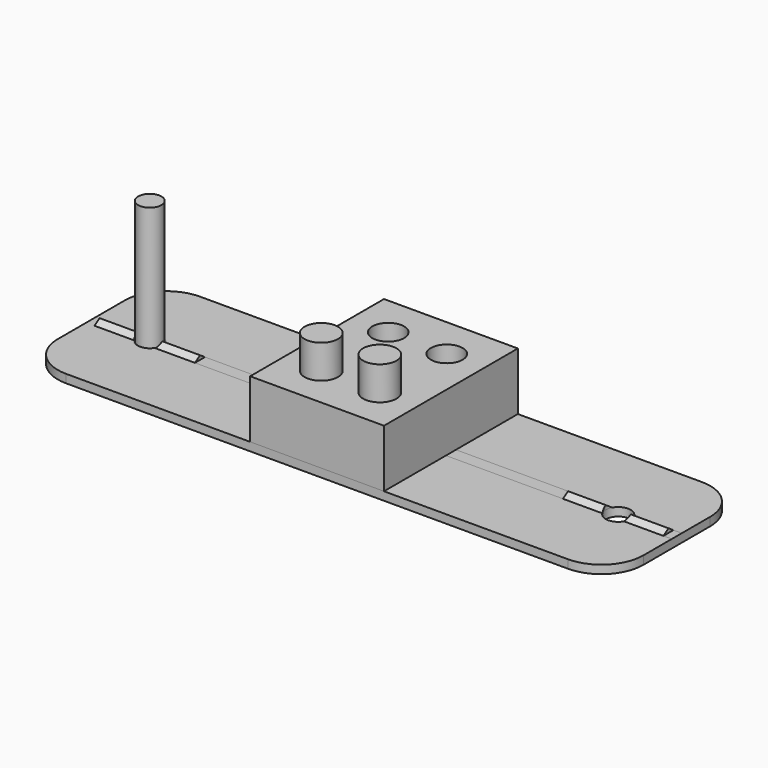
from build123d import *
from build123d import SkipClean  # not in build123d's __all__

# Parameters (mm, degrees)
F0_W      = 70
F0_H      = 20
F1_DEPTH  = 1
F3_D      = 3
F4_R      = 5
F7_DEPTH  = 0.5
F9_DEPTH  = 69.001
F10_W     = 16
F10_H     = 9.25
F10_H_2   = 1.5
F11_DEPTH = 6.9
F12_R     = 1.9
F13_DEPTH = 4.5
F14_R     = 2
F15_DEPTH = 4
F16_R     = 1.5
F17_DEPTH = 1
F18_R     = 1.4
F19_DEPTH = 14.8


with BuildPart() as f1:
    # F0 (on Top) → F1 (new body)
    with BuildSketch(Plane.XY):
        Rectangle(F0_W, F0_H)
    extrude(amount=F1_DEPTH)

    # F3 (through all)
    with Locations(Plane.XY.offset(1)):
        with Locations((-28, 0), (28, 0)):
            Hole(F3_D / 2)

    # F4
    f4_edges = [f1.edges().sort_by_distance(p)[0] for p in [
        (-35, 10, 0.5),
        (-35, -10, 0.5),
        (35, 10, 0.5),
        (35, -10, 0.5),
    ]]
    fillet(f4_edges, radius=F4_R)

    # F5 (on face) + F6 (on face) → F7 (join)
    with BuildSketch(Plane.XY.offset(1)):
        with BuildLine():
            Line((-29.2990381057, 0.75), (-34, 0.75))
            Line((-34, 0.75), (-34, -0.75))
            Line((-34, -0.75), (-29.2990381057, -0.75))
            ThreePointArc((-29.2990381057, -0.75), (-29.5, 0), (-29.2990381057, 0.75))
        make_face()
        with BuildLine():
            Line((-22, 0.75), (-26.7009618943, 0.75))
            ThreePointArc((-26.7009618943, 0.75), (-26.5511112606, 0.3882285677), (-26.5, 0))
            ThreePointArc((-26.5, 0), (-26.5511112606, -0.3882285677), (-26.7009618943, -0.75))
            Line((-26.7009618943, -0.75), (-22, -0.75))
            Line((-22, -0.75), (-22, 0.75))
        make_face()
    with BuildSketch(Plane.XY.offset(1)):
        with BuildLine():
            Line((26.7009618943, 0.75), (22, 0.75))
            Line((22, 0.75), (22, -0.75))
            Line((22, -0.75), (26.7009618943, -0.75))
            ThreePointArc((26.7009618943, -0.75), (26.5, 0), (26.7009618943, 0.75))
        make_face()
        with BuildLine():
            Line((34, 0.75), (29.2990381057, 0.75))
            ThreePointArc((29.2990381057, 0.75), (29.4488887394, 0.3882285677), (29.5, 0))
            ThreePointArc((29.5, 0), (29.4488887394, -0.3882285677), (29.2990381057, -0.75))
            Line((29.2990381057, -0.75), (34, -0.75))
            Line((34, -0.75), (34, 0.75))
        make_face()
    with SkipClean():  # cleaning this boolean's faces spoils the solid; the shape is the same uncleaned
        extrude(amount=F7_DEPTH)

    # F8 (on face) → F9 (cut, through all)
    with BuildSketch(Plane(origin=(-34, 0, 0), x_dir=(0, -1, 0), z_dir=(-1, 0, 0))):
        Polygon((-0.75, 1.5), (-0.75, 1), (0, 1.5), align=None)
        Polygon((0.75, 1.5), (0, 1.5), (0.75, 1), align=None)
    with SkipClean():  # cleaning this boolean's faces spoils the solid; the shape is the same uncleaned
        extrude(amount=-F9_DEPTH, mode=Mode.SUBTRACT)

    # F10 (on face) → F11 (join)
    with BuildSketch(Plane.XY.offset(1)):
        with Locations((0, -5.375)):
            Rectangle(F10_W, F10_H)
        Rectangle(F10_W, F10_H_2)
        with Locations((0, 5.375)):
            Rectangle(F10_W, F10_H)
    with SkipClean():  # cleaning this boolean's faces spoils the solid; the shape is the same uncleaned
        extrude(amount=F11_DEPTH)

    # F12 (on face) → F13 (cut)
    with BuildSketch(Plane.XY.offset(7.9)):
        with Locations((-3.5, 5)):
            Circle(F12_R)
        with Locations((3.5, 5)):
            Circle(F12_R)
    with SkipClean():  # cleaning this boolean's faces spoils the solid; the shape is the same uncleaned
        extrude(amount=-F13_DEPTH, mode=Mode.SUBTRACT)

    # F14 (on face) → F15 (join)
    with BuildSketch(Plane.XY.offset(7.9)):
        with Locations((-3.5, -5)):
            Circle(F14_R)
        with Locations((3.5, -5)):
            Circle(F14_R)
    with SkipClean():  # cleaning this boolean's faces spoils the solid; the shape is the same uncleaned
        extrude(amount=F15_DEPTH)

    # F16 (on face) → F17 (join)
    with BuildSketch(Plane.XY.offset(1)):
        with Locations((-28, 0)):
            Circle(F16_R)
    with SkipClean():  # cleaning this boolean's faces spoils the solid; the shape is the same uncleaned
        extrude(amount=-F17_DEPTH)

    # F18 (on face) → F19 (join)
    with BuildSketch(Plane.XY.offset(1)):
        with Locations((-28, 0)):
            Circle(F18_R)
    with SkipClean():  # cleaning this boolean's faces spoils the solid; the shape is the same uncleaned
        extrude(amount=F19_DEPTH)


solid = f1.part
